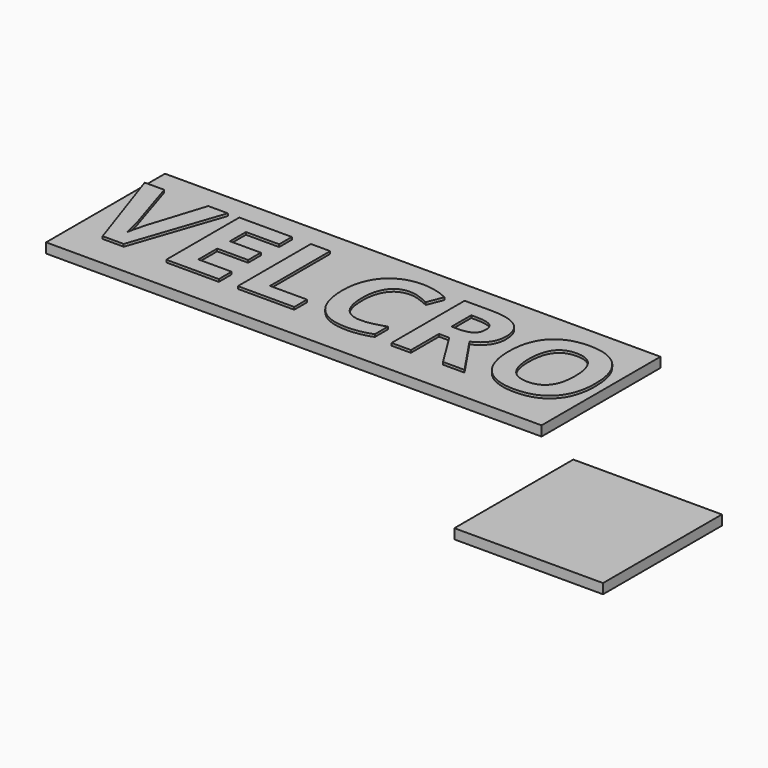
from build123d import *

# Parameters (mm, degrees)
F0_W         = 30
F0_H         = 30
F1_DEPTH     = 2
F0_W_2       = 100
F2_TEXT_SIZE = 25.8074922376
F3_DEPTH     = 0.5


# Not quite as in the source:
# - Text() gives the source's letters only with a copy of the font that has no kerning and outlines rounded to 1/6400 em; it was checked with that copy


with BuildPart() as f1:
    # F0 (on Top) → F1 (new body)
    with BuildSketch(Plane.XY):
        Rectangle(F0_W, F0_H)
    extrude(amount=F1_DEPTH)


with BuildPart() as f1b:
    # F0 (on Top) → F1, piece 2 (new body)
    with BuildSketch(Plane.XY):
        with Locations((-76.1964015663, 35.9865700454)):
            Rectangle(F0_W_2, F0_H)
    extrude(amount=F1_DEPTH)

    # F2 (on face) → F3 (join)
    with BuildSketch(Plane.XY.offset(2)):
        with Locations((-126.1964015663, 27.4428119761)):
            Text('VELCRO', F2_TEXT_SIZE, font='Open Sans', font_style=FontStyle.BOLD, text_align=(TextAlign.LEFT, TextAlign.BOTTOM))
    extrude(amount=F3_DEPTH)


solid = Compound([f1.part, f1b.part])
